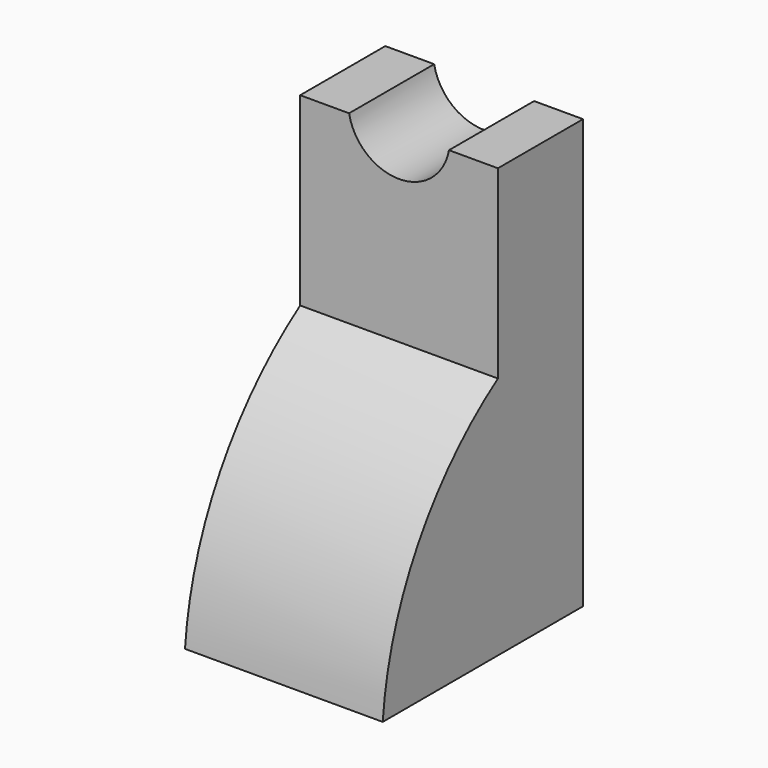
from build123d import *

# Parameters (mm, degrees)
F1_DEPTH    = 11
F2_W        = 20.4476909052
F2_H        = 25.2064025609
F3_DEPTH    = 15
F4_T1_DEPTH = 160.2446021291


# Not quite as in the source:
# - a fillet or chamfer that OpenCascade refuses, or shapes differently, is made with other operations: its cross-section is extruded or revolved along the edge and cut away or added


with BuildPart() as f1:
    # F0 (on Front) → F1 (new body)
    with BuildSketch(Plane.XZ):
        with BuildLine():
            Line((-10.2238454526, -37.989632494), (10.2238454526, -37.989632494))
            Line((10.2238454526, -37.989632494), (10.2238454526, 6.3570427475))
            Line((10.2238454526, 6.3570427475), (5.1648352034, 6.3570427475))
            ThreePointArc((5.1648352034, 6.3570427475), (0, 2.048837482), (-5.1648352034, 6.3570427475))
            Line((-5.1648352034, 6.3570427475), (-10.2238454526, 6.3570427475))
            Line((-10.2238454526, 6.3570427475), (-10.2238454526, -37.989632494))
        make_face()
    extrude(amount=F1_DEPTH)

    # F2 (on face) → F3 (join)
    with BuildSketch(Plane.XZ.offset(11)):
        with Locations((0, -25.3864312136)):
            Rectangle(F2_W, F2_H)
    extrude(amount=F3_DEPTH)

    # F4: fillet of radius 33.557568517 on 1 edges, made by hand

    # F4_s2 → F4_t1 (cut)
    with BuildSketch(Plane.YZ.offset(-80.1223010645)):
        with BuildLine():
            ThreePointArc((-26, -40.7426121779), (-22.0131710898, -24.8781309737), (-11, -12.7832299331))
            Line((-11, -12.7832299331), (-26, -12.7832299331))
            Line((-26, -12.7832299331), (-26, -40.7426121779))
        make_face()
    extrude(amount=F4_T1_DEPTH, mode=Mode.SUBTRACT)


solid = f1.part
